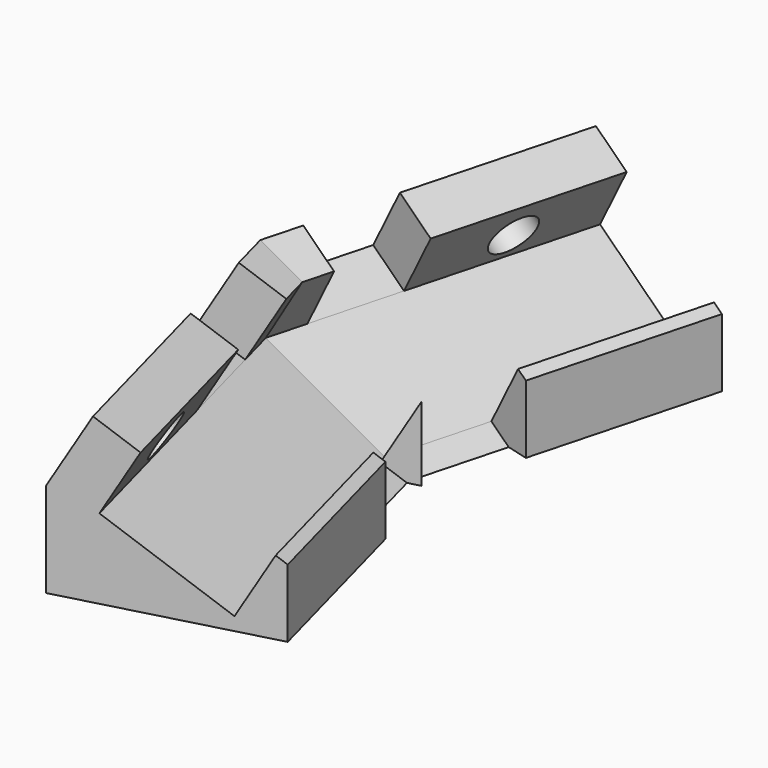
from build123d import *

# Parameters (mm, degrees)
F1_DEPTH       = 20
F4_REACH       = 59.8904911491
F6_REACH       = 49.0077165035
F8_DEPTH       = 17.7213446758
F8_DEPTH_BACK  = 25
F10_REACH      = 31.5666498146
F12_DEPTH      = 19.1713446758
F12_DEPTH_BACK = 31.9213446758
F13_R          = 2.5
F14_DEPTH      = 5


with BuildPart() as f1:
    # F0 (on Top) → F1 (new body)
    with BuildSketch(Plane.XY):
        Polygon((7.7645713531, -28.9777747887), (0, 0), (7.7645713531, 28.9777747887), (-13.4857968253, 34.6717937809), (-22.776075969, 0), (-13.4857968253, -34.6717937809), align=None)
    extrude(amount=F1_DEPTH)

    f4_end = Plane(origin=(0, 0, 20), x_dir=(0, 0, 1), z_dir=(0, 1, 0))
    # F3 (on face) → F4 (cut, up to a plane its end follows)
    with BuildSketch(Plane(origin=(7.7645713531, -28.9777747887, 0), x_dir=(0.9659258263, 0.2588190451, 0), z_dir=(0.2588190451, -0.9659258263, 0))):
        Polygon((-13.3987803669, 15), (-17.1487803669, 8.5048094716), (-4.8512196331, 1.4048094716), (-1.1012196331, 7.9), (0, 7.9), (0, 20), (-13.3987803669, 20), align=None)
    f4_long = extrude(amount=-F4_REACH, mode=Mode.PRIVATE)
    add(split(f4_long, bisect_by=f4_end, keep=Keep.BOTTOM, mode=Mode.PRIVATE), mode=Mode.SUBTRACT)

    f6_end = Plane(origin=(0, 0, 20), x_dir=(0, 0, 1), z_dir=(0, 1, 0))
    # F5 (on face) → F6 (cut, up to a plane its end follows)
    with BuildSketch(Plane(origin=(7.7645713531, -28.9777747887, 0), x_dir=(0.9659258263, 0.2588190451, 0), z_dir=(0.2588190451, -0.9659258263, 0))):
        Polygon((-22, 20), (-22, 10.1022505884), (-17.7289073858, 17.5), (-13.3987803669, 15), (-13.3987803669, 20), align=None)
    f6_long = extrude(amount=-F6_REACH, mode=Mode.PRIVATE)
    add(split(f6_long, bisect_by=f6_end, keep=Keep.BOTTOM, mode=Mode.PRIVATE), mode=Mode.SUBTRACT)

    # F7 (on face) → F8 (cut, two sides)
    with BuildSketch(Plane(origin=(-15.9805432759, -4.2819736654, 9.5518420887), x_dir=(-0.1923952931, 0.9745560663, 0.1149979338), z_dir=(0.8365163037, 0.224143868, -0.5))) as f8_sk:
        Polygon((-28.8989639862, 10.218925907), (-36.8281195036, 11.2812313158), (-37.8240308243, 3.8476480182), (-29.8948753069, 2.7853426095), align=None)
    extrude(amount=-F8_DEPTH, mode=Mode.SUBTRACT)
    extrude(f8_sk.sketch, amount=F8_DEPTH_BACK, mode=Mode.SUBTRACT)

    f10_end = Plane(origin=(0, 0, 20), x_dir=(0, 0, 1), z_dir=(0, 1, 0))
    # F9 (on face) → F10 (cut, up to a plane its end follows)
    with BuildSketch(Plane(origin=(7.7645713531, -28.9777747887, 0), x_dir=(0.9659258263, 0.2588190451, 0), z_dir=(0.2588190451, -0.9659258263, 0))):
        Polygon((0, 7.9), (-1.1012196331, 7.9), (0, 7.2642105484), align=None)
    f10_long = extrude(amount=-F10_REACH, mode=Mode.PRIVATE)
    add(split(f10_long, bisect_by=f10_end, keep=Keep.BOTTOM, mode=Mode.PRIVATE), mode=Mode.SUBTRACT)

    # F11 (on face) → F12 (cut, two sides)
    with BuildSketch(Plane(origin=(-4.1020117628, -1.0991307392, 2.4518420887), x_dir=(0.1923952931, -0.9745560663, -0.1149979338), z_dir=(-0.8365163037, -0.224143868, 0.5))) as f12_sk:
        Polygon((8.7836172997, 7.5239804569), (-1.127827097, 6.196098696), (-0.1319157763, -1.2374846015), (9.7795286204, 0.0903971594), align=None)
    extrude(amount=-F12_DEPTH, mode=Mode.SUBTRACT)
    extrude(f12_sk.sketch, amount=F12_DEPTH_BACK, mode=Mode.SUBTRACT)

    # F13 (on face) → F14 (cut, through all)
    with BuildSketch(Plane(origin=(-20.1631247946, -5.4026930056, 12.0518420887), x_dir=(0.1923952931, -0.9745560663, -0.1149979338), z_dir=(-0.8365163037, -0.224143868, 0.5))):
        with Locations((19.4084412411, 4.6381834861)):
            Circle(F13_R)
    extrude(amount=-F14_DEPTH, mode=Mode.SUBTRACT)

    # F15: F1 across plane


with BuildPart() as f1_1:
    add(f1.part)
    add(f1.part.mirror(Plane.XZ), mode=Mode.INTERSECT)


solid = f1_1.part
